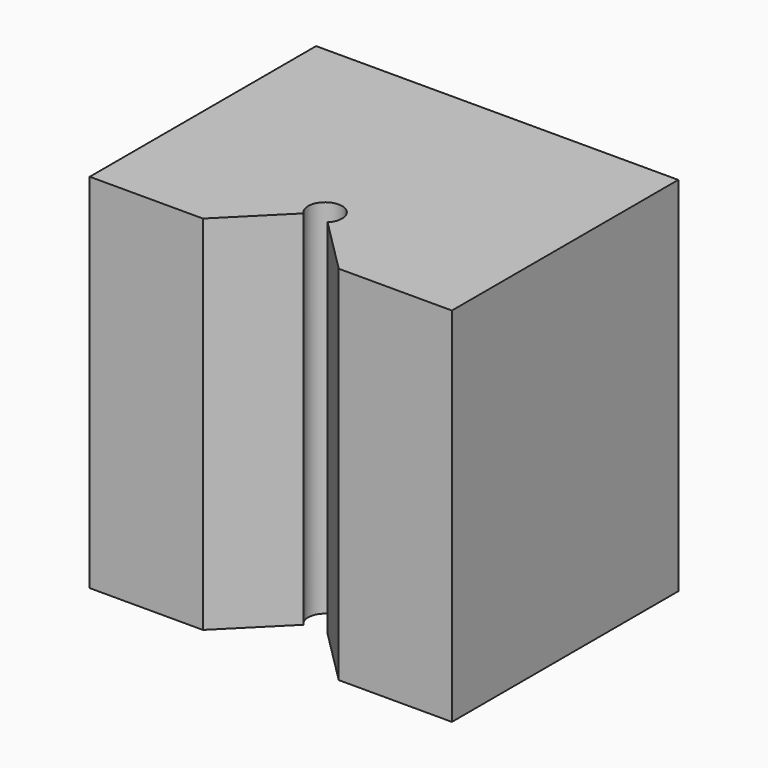
from build123d import *

# Parameters (mm, degrees)
F0_W     = 32
F0_H     = 32
F1_DEPTH = 25
F3_DEPTH = 32.001


with BuildPart() as f1:
    # F0 (on Front) → F1 (new body)
    with BuildSketch(Plane.XZ):
        Rectangle(F0_W, F0_H)
    extrude(amount=-F1_DEPTH)

    # F2 (on face) → F3 (cut, through all)
    with BuildSketch(Plane.XY.offset(16)):
        with BuildLine():
            Line((-1.0606601718, 4.9393398282), (-6, 0))
            Line((-6, 0), (6, 0))
            Line((6, 0), (1.0606601718, 4.9393398282))
            ThreePointArc((1.0606601718, 4.9393398282), (0, 4.5), (-1.0606601718, 4.9393398282))
        make_face()
        with BuildLine():
            ThreePointArc((1.5, 6), (-0.5740251485, 7.3858192988), (-1.0606601718, 4.9393398282))
            Line((-1.0606601718, 4.9393398282), (0, 6))
            Line((0, 6), (1.0606601718, 4.9393398282))
            ThreePointArc((1.0606601718, 4.9393398282), (1.3858192988, 5.4259748515), (1.5, 6))
        make_face()
        with BuildLine():
            Line((0, 6), (-1.0606601718, 4.9393398282))
            ThreePointArc((-1.0606601718, 4.9393398282), (0, 4.5), (1.0606601718, 4.9393398282))
            Line((1.0606601718, 4.9393398282), (0, 6))
        make_face()
    extrude(amount=-F3_DEPTH, mode=Mode.SUBTRACT)


solid = f1.part
